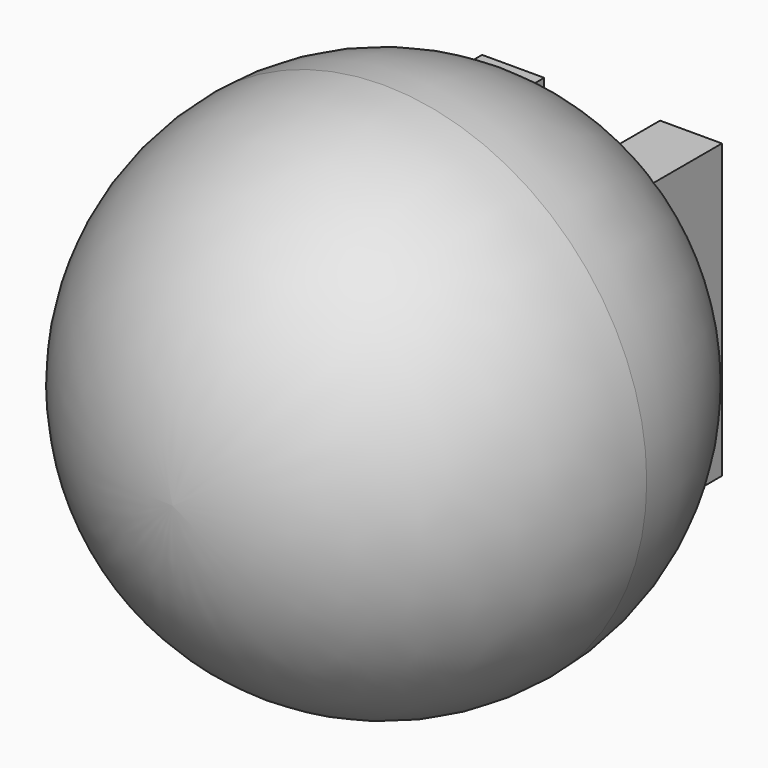
from build123d import *

# Parameters (mm, degrees)
F0_R         = 19.05
F1_DEPTH     = 38.1
F2_R         = 19.04999
F3_TEXT_SIZE = 29.6496734437
F4_DEPTH     = 25.4


# Not quite as in the source:
# - a fillet or chamfer is up to 0.001 mm smaller than in the source, because OpenCascade refuses the exact size
# - Text() gives the source's letters only with a copy of the font that has no kerning and outlines rounded to 1/6400 em; it was checked with that copy


with BuildPart() as f1:
    # F0 (on Front) → F1 (new body)
    with BuildSketch(Plane.XZ):
        with Locations((-17.1134956181, 21.2595481426)):
            Circle(F0_R)
    extrude(amount=F1_DEPTH)

    # F2 (radius 19.05 in the source; OpenCascade refuses exactly that, so slightly less here)
    f2_edges = [f1.edges().sort_by_distance(p)[0] for p in [
        (-36.163496, 0, 21.259548),
        (-36.163496, -38.1, 21.259548),
    ]]
    fillet(f2_edges, radius=F2_R)

    # F3 (on Front) → F4 (join)
    with BuildSketch(Plane.XZ):
        with Locations((-27.8755929321, 10.6738805771)):
            Text('H', F3_TEXT_SIZE, font='Open Sans', font_style=FontStyle.BOLD, text_align=(TextAlign.LEFT, TextAlign.BOTTOM))
    extrude(amount=F4_DEPTH)


solid = f1.part
